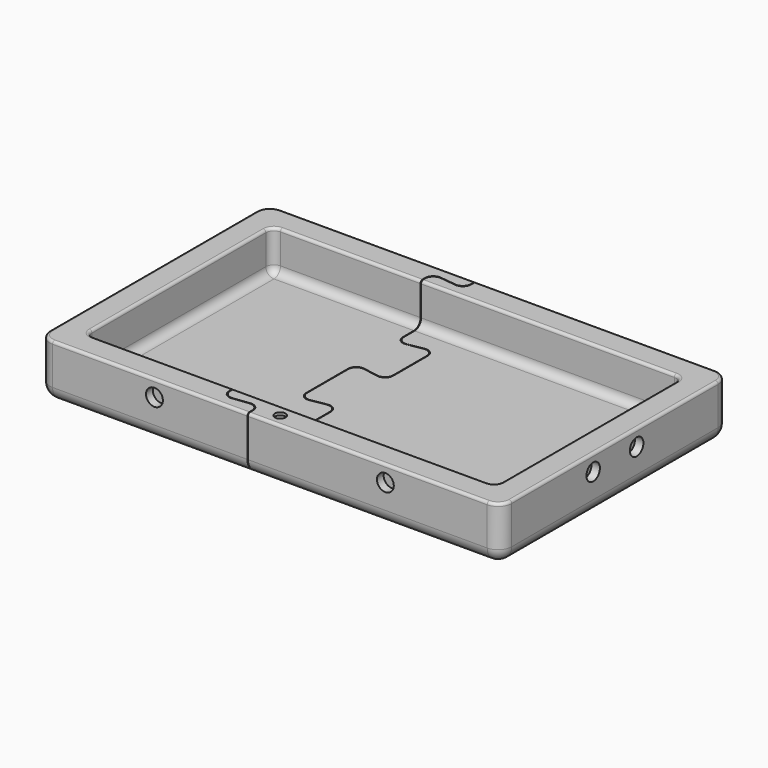
from build123d import *

# Parameters (mm, degrees)
F0_W      = 170
F0_H      = 105
F0_R      = 2
F1_DEPTH  = 20
F2_DEPTH  = 15
F3_R      = 5
F4_R      = 3
F5_R      = 1
F6_R      = 3.1
F7_DEPTH  = 3.1
F8_R      = 3.1
F9_DEPTH  = 3.1
F10_R     = 3.1
F11_DEPTH = 3.1
F12_R     = 3.1
F13_DEPTH = 3.1
F14_DEPTH = 1
F15_ANGLE = 180
F17_DEPTH = 25
F18_DEPTH = 25


# Not quite as in the source:
# - a feature names something its author has since deleted; it is built from what else it names


with BuildPart() as f1:
    # F0 (on Top) → F1 (new body)
    with BuildSketch(Plane.XY):
        Rectangle(F0_W, F0_H)
        with Locations((0, -47.75)):
            Circle(F0_R, mode=Mode.SUBTRACT)
        with BuildLine():
            ThreePointArc((-75.5, 40), (-74.6213203436, 42.1213203436), (-72.5, 43))
            Line((-72.5, 43), (72.5, 43))
            ThreePointArc((72.5, 43), (74.6213203436, 42.1213203436), (75.5, 40))
            Line((75.5, 40), (75.5, -40))
            ThreePointArc((75.5, -40), (74.6213203436, -42.1213203436), (72.5, -43))
            Line((72.5, -43), (-72.5, -43))
            ThreePointArc((-72.5, -43), (-74.6213203436, -42.1213203436), (-75.5, -40))
            Line((-75.5, -40), (-75.5, 40))
        make_face(mode=Mode.SUBTRACT)
        with BuildLine():
            Line((72.5, 43), (-72.5, 43))
            ThreePointArc((-72.5, 43), (-74.6213203436, 42.1213203436), (-75.5, 40))
            Line((-75.5, 40), (-75.5, -40))
            ThreePointArc((-75.5, -40), (-74.6213203436, -42.1213203436), (-72.5, -43))
            Line((-72.5, -43), (72.5, -43))
            ThreePointArc((72.5, -43), (74.6213203436, -42.1213203436), (75.5, -40))
            Line((75.5, -40), (75.5, 40))
            ThreePointArc((75.5, 40), (74.6213203436, 42.1213203436), (72.5, 43))
        make_face()
        with Locations((0, -47.75)):
            Circle(F0_R)
    extrude(amount=F1_DEPTH)

    # F0 (on Top) → F2 (cut)
    with BuildSketch(Plane.XY):
        with BuildLine():
            Line((72.5, 43), (-72.5, 43))
            ThreePointArc((-72.5, 43), (-74.6213203436, 42.1213203436), (-75.5, 40))
            Line((-75.5, 40), (-75.5, -40))
            ThreePointArc((-75.5, -40), (-74.6213203436, -42.1213203436), (-72.5, -43))
            Line((-72.5, -43), (72.5, -43))
            ThreePointArc((72.5, -43), (74.6213203436, -42.1213203436), (75.5, -40))
            Line((75.5, -40), (75.5, 40))
            ThreePointArc((75.5, 40), (74.6213203436, 42.1213203436), (72.5, 43))
        make_face()
    extrude(amount=F2_DEPTH, mode=Mode.SUBTRACT)

    # F3
    f3_edges = [f1.edges().sort_by_distance(p)[0] for p in [
        (0, 52.5, 20),
        (-85, 0, 20),
        (0, -52.5, 20),
        (85, 0, 20),
        (85, 52.5, 10),
        (-85, 52.5, 10),
        (-85, -52.5, 10),
        (85, -52.5, 10),
    ]]
    fillet(f3_edges, radius=F3_R)

    # F4
    f4_edges = [f1.edges().sort_by_distance(p)[0] for p in [
        (0, 43, 15),
        (-74.62132, 42.12132, 15),
        (-75.5, 0, 15),
        (-74.62132, -42.12132, 15),
        (0, -43, 15),
        (74.62132, -42.12132, 15),
        (75.5, 0, 15),
        (74.62132, 42.12132, 15),
    ]]
    fillet(f4_edges, radius=F4_R)

    # F5
    f5_edges = [f1.edges().sort_by_distance(p)[0] for p in [
        (0, 52.5, 0),
        (83.535534, 51.035534, 0),
        (-83.535534, 51.035534, 0),
        (85, 0, 0),
        (-85, 0, 0),
        (83.535534, -51.035534, 0),
        (-83.535534, -51.035534, 0),
        (0, -52.5, 0),
        (0, 43, 0),
        (-74.62132, 42.12132, 0),
        (-75.5, 0, 0),
        (-74.62132, -42.12132, 0),
        (0, -43, 0),
        (74.62132, -42.12132, 0),
        (75.5, 0, 0),
        (74.62132, 42.12132, 0),
    ]]
    fillet(f5_edges, radius=F5_R)

    # F6 (on face) → F7 (cut)
    with BuildSketch(Plane.XZ.offset(52.5)):
        with Locations((42.5, 6)):
            Circle(F6_R)
        with Locations((-42.5, 6)):
            Circle(F6_R)
    extrude(amount=-F7_DEPTH, mode=Mode.SUBTRACT)

    # F8 (on face) → F9 (cut)
    with BuildSketch(Plane(origin=(0, 52.5, 0), x_dir=(-1, 0, 0), z_dir=(0, 1, 0))):
        with Locations((42.5, 6)):
            Circle(F8_R)
        with Locations((-42.5, 6)):
            Circle(F8_R)
    extrude(amount=-F9_DEPTH, mode=Mode.SUBTRACT)

    # F10 (on face) → F11 (cut)
    with BuildSketch(Plane(origin=(-85, 0, 0), x_dir=(0, -1, 0), z_dir=(-1, 0, 0))):
        with Locations((10, 6)):
            Circle(F10_R)
        with Locations((-10, 6)):
            Circle(F10_R)
    extrude(amount=-F11_DEPTH, mode=Mode.SUBTRACT)

    # F12 (on face) → F13 (cut)
    with BuildSketch(Plane.YZ.offset(85)):
        with Locations((10, 6)):
            Circle(F12_R)
        with Locations((-10, 6)):
            Circle(F12_R)
    extrude(amount=-F13_DEPTH, mode=Mode.SUBTRACT)

    # F0 (on Top) → F14 (cut)
    with BuildSketch(Plane.XY):
        with Locations((0, -47.75)):
            Circle(F0_R)
    extrude(amount=F14_DEPTH, mode=Mode.SUBTRACT)


with BuildPart() as f1_1:
    # F15: moved
    add(f1.part.rotate(Axis((0, 0, 0), (0, 1, 0)), F15_ANGLE))


with BuildPart() as f17:
    # F16 (on Top) → F17 (new body)
    with BuildSketch(Plane.XY):
        with BuildLine():
            Line((-20.9563169628, -9.6620759565), (-20.9563169628, 0))
            Line((-20.9563169628, 0), (-20.9563169628, 9.6620759565))
            ThreePointArc((-20.9563169628, 9.6620759565), (-19.8846797919, 11.9602092859), (-17.4353724298, 12.6164992155))
            Line((-17.4353724298, 12.6164992155), (-11.8024505631, 11.6232631102))
            ThreePointArc((-11.8024505631, 11.6232631102), (-9.3531432011, 12.2795530399), (-8.2815060301, 14.5776863693))
            Line((-8.2815060301, 14.5776863693), (-8.2815060301, 29.9721352199))
            ThreePointArc((-8.2815060301, 29.9721352199), (-9.3531432011, 32.2702685493), (-11.8024505631, 32.926558479))
            Line((-11.8024505631, 32.926558479), (-17.4353724298, 31.9333223736))
            ThreePointArc((-17.4353724298, 31.9333223736), (-19.8846797919, 32.5896123033), (-20.9563169628, 34.8877456327))
            Line((-20.9563169628, 34.8877456327), (-20.9563169628, 45.1240298712))
            ThreePointArc((-20.9563169628, 45.1240298712), (-19.9490884736, 47.3665422359), (-17.6037424924, 48.1032397065))
            Line((-17.6037424924, 48.1032397065), (-11.6340805006, 47.3967602935))
            ThreePointArc((-11.6340805006, 47.3967602935), (-9.2887345193, 48.1334577641), (-8.2815060301, 50.3759701288))
            Line((-8.2815060301, 50.3759701288), (-8.2815060301, 69.1191965569))
            Line((-8.2815060301, 69.1191965569), (-109.5252448242, 69.1191965569))
            Line((-109.5252448242, 69.1191965569), (-109.5252448242, 0))
            Line((-109.5252448242, 0), (-109.5252448242, -69.1191965569))
            Line((-109.5252448242, -69.1191965569), (-8.2815060301, -69.1191965569))
            Line((-8.2815060301, -69.1191965569), (-8.2815060301, -50.3759701288))
            ThreePointArc((-8.2815060301, -50.3759701288), (-9.2887345193, -48.1334577641), (-11.6340805006, -47.3967602935))
            Line((-11.6340805006, -47.3967602935), (-17.6037424924, -48.1032397065))
            ThreePointArc((-17.6037424924, -48.1032397065), (-19.9490884736, -47.3665422359), (-20.9563169628, -45.1240298712))
            Line((-20.9563169628, -45.1240298712), (-20.9563169628, -34.8877456327))
            ThreePointArc((-20.9563169628, -34.8877456327), (-19.8846797919, -32.5896123033), (-17.4353724298, -31.9333223736))
            Line((-17.4353724298, -31.9333223736), (-11.8024505631, -32.926558479))
            ThreePointArc((-11.8024505631, -32.926558479), (-9.3531432011, -32.2702685493), (-8.2815060301, -29.9721352199))
            Line((-8.2815060301, -29.9721352199), (-8.2815060301, -14.5776863693))
            ThreePointArc((-8.2815060301, -14.5776863693), (-9.3531432011, -12.2795530399), (-11.8024505631, -11.6232631102))
            Line((-11.8024505631, -11.6232631102), (-17.4353724298, -12.6164992155))
            ThreePointArc((-17.4353724298, -12.6164992155), (-19.8846797919, -11.9602092859), (-20.9563169628, -9.6620759565))
        make_face()
    extrude(amount=-F17_DEPTH)


with BuildPart() as f18:
    # F16 (on Top) → F18 (new body)
    with BuildSketch(Plane.XY):
        with BuildLine():
            Line((105.8235841181, 69.1191965569), (-8.0815060301, 69.1191965569))
            Line((-8.0815060301, 69.1191965569), (-8.0815060301, 50.1509054536))
            ThreePointArc((-8.0815060301, 50.1509054536), (-9.0887345193, 47.9083930889), (-11.4340805006, 47.1716956182))
            Line((-11.4340805006, 47.1716956182), (-17.4037424924, 47.8781750312))
            ThreePointArc((-17.4037424924, 47.8781750312), (-19.7490884736, 47.1414775606), (-20.7563169628, 44.8989651959))
            Line((-20.7563169628, 44.8989651959), (-20.7563169628, 35.1260963512))
            ThreePointArc((-20.7563169628, 35.1260963512), (-19.6846797919, 32.8279630218), (-17.2353724298, 32.1716730922))
            Line((-17.2353724298, 32.1716730922), (-11.6024505631, 33.1649091975))
            ThreePointArc((-11.6024505631, 33.1649091975), (-9.1531432011, 32.5086192678), (-8.0815060301, 30.2104859384))
            Line((-8.0815060301, 30.2104859384), (-8.0815060301, 14.3393356507))
            ThreePointArc((-8.0815060301, 14.3393356507), (-9.1531432011, 12.0412023214), (-11.6024505631, 11.3849123917))
            Line((-11.6024505631, 11.3849123917), (-17.2353724298, 12.378148497))
            ThreePointArc((-17.2353724298, 12.378148497), (-19.6846797919, 11.7218585673), (-20.7563169628, 9.423725238))
            Line((-20.7563169628, 9.423725238), (-20.7563169628, 0))
            Line((-20.7563169628, 0), (-20.7563169628, -9.423725238))
            ThreePointArc((-20.7563169628, -9.423725238), (-19.6846797919, -11.7218585673), (-17.2353724298, -12.378148497))
            Line((-17.2353724298, -12.378148497), (-11.6024505631, -11.3849123917))
            ThreePointArc((-11.6024505631, -11.3849123917), (-9.1531432011, -12.0412023214), (-8.0815060301, -14.3393356507))
            Line((-8.0815060301, -14.3393356507), (-8.0815060301, -30.2104859384))
            ThreePointArc((-8.0815060301, -30.2104859384), (-9.1531432011, -32.5086192678), (-11.6024505631, -33.1649091975))
            Line((-11.6024505631, -33.1649091975), (-17.2353724298, -32.1716730922))
            ThreePointArc((-17.2353724298, -32.1716730922), (-19.6846797919, -32.8279630218), (-20.7563169628, -35.1260963512))
            Line((-20.7563169628, -35.1260963512), (-20.7563169628, -44.8989651959))
            ThreePointArc((-20.7563169628, -44.8989651959), (-19.7490884736, -47.1414775606), (-17.4037424924, -47.8781750312))
            Line((-17.4037424924, -47.8781750312), (-11.4340805006, -47.1716956182))
            ThreePointArc((-11.4340805006, -47.1716956182), (-9.0887345193, -47.9083930889), (-8.0815060301, -50.1509054536))
            Line((-8.0815060301, -50.1509054536), (-8.0815060301, -69.1191965569))
            Line((-8.0815060301, -69.1191965569), (105.8235841181, -69.1191965569))
            Line((105.8235841181, -69.1191965569), (105.8235841181, 69.1191965569))
        make_face()
    extrude(amount=-F18_DEPTH)


with BuildPart() as f19_1:
    # F19: copy of F1
    add(f1_1.part)


with BuildPart() as f1_2:
    add(f1_1.part)

    # F20: intersect F17
    add(f17.part, mode=Mode.INTERSECT)


with BuildPart() as f18_1:
    add(f18.part)

    # F21: intersect F19_1
    add(f19_1.part, mode=Mode.INTERSECT)


solid = Compound([f1_2.part, f18_1.part])
